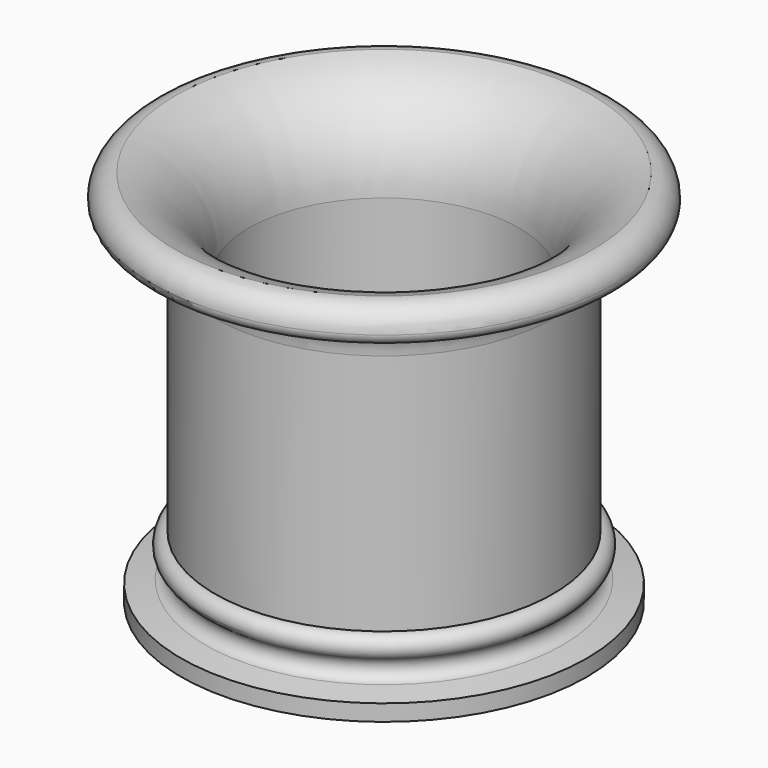
from build123d import *


# Not quite as in the source:
# - ends of sketch curves that miss each other by under 0.0002 mm in the source are joined


with BuildPart() as f2:
    # F0 (on Front) → F2 (revolve)
    with BuildSketch(Plane.XZ):
        with BuildLine():
            Line((-45.72, -21.8209084123), (-38.1, -21.8209084123))
            Line((-38.1, -21.8209084123), (-30.48, -21.8209084123))
            Line((-30.48, -21.8209084123), (0, -21.8209084123))
            Line((0, -21.8209084123), (0, -14.2009084123))
            Line((0, -14.2009084123), (-24.13, -14.2009084123))
            ThreePointArc((-24.13, -14.2009084123), (-28.6201280605, -12.3410364729), (-30.48, -7.8509084123))
            Line((-30.48, -7.8509084123), (-30.48, 42.4047588836))
            ThreePointArc((-30.48, 42.4047588836), (-35.1108174237, 55.7111992459), (-47.0022115332, 63.2676912401))
            ThreePointArc((-47.0022115332, 63.2676912401), (-50.5890500932, 61.7769207718), (-52.0740705111, 58.1876977634))
            ThreePointArc((-52.0740705111, 58.1876977634), (-51.3301217353, 56.3916498008), (-49.5340705111, 55.647701025))
            Line((-49.5340705111, 55.647701025), (-46.99, 55.647701025))
            ThreePointArc((-46.99, 55.647701025), (-40.7038207153, 53.0438803098), (-38.1, 46.757701025))
            Line((-38.1, 46.757701025), (-38.1, -7.8458491338))
            ThreePointArc((-38.1, -7.8458491338), (-40.5534515988, -9.7284487592), (-39.37, -12.5855536594))
            ThreePointArc((-39.37, -12.5855536594), (-38.1434137036, -15.2528657816), (-40.2521623329, -17.2954737024))
            Line((-40.2521623329, -17.2954737024), (-45.72, -18.1402750313))
            Line((-45.72, -18.1402750313), (-45.72, -21.8209084123))
        make_face()
    revolve(axis=Axis((0, 0, 8.5881464183), (0, 0, -1)))


solid = f2.part
